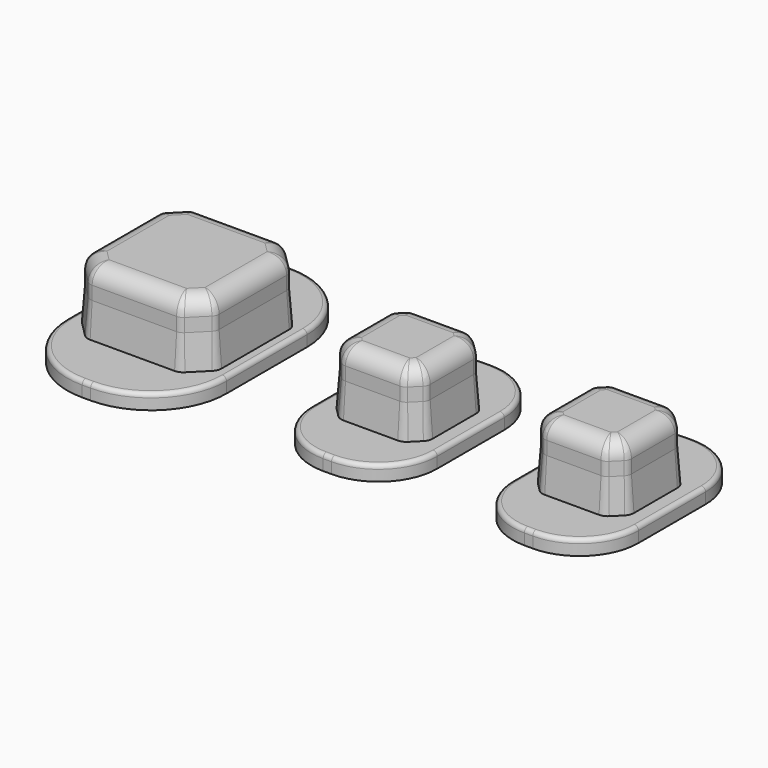
from build123d import *

# Parameters (mm, degrees)
F0_W        = 9.5
F0_H        = 15
F1_DEPTH    = 0.9
F0_W_2      = 7.5
F0_H_2      = 12
F3_DEPTH    = 3.8
F5_DEPTH    = 3.8
F6_R        = 4.5
F7_R        = 3.5
F8_SIZE     = 1.2
F9_SIZE     = 0.8
F10_R       = 1
F10_2_R     = 1
F11_R       = 0.5
F11_2_R     = 0.5
F12_SIZE2   = 2
F12_SIZE    = 0.15
F12_2_SIZE2 = 2
F12_2_SIZE  = 0.15
F14_R       = 0.25
F14_2_R     = 0.25
F14_3_R     = 0.25


with BuildPart() as f1:
    # F0 (on Top) → F1 (new body)
    with BuildSketch(Plane.XY):
        with Locations((-18.6926795918, 4.292611382)):
            Rectangle(F0_W, F0_H)
    extrude(amount=F1_DEPTH)

    # F2 (on face) → F3 (join)
    with BuildSketch(Plane.XY.offset(0.9)):
        Polygon((-14.7676795918, 8.217611382), (-22.6176795918, 8.217611382), (-22.6176795918, 4.292611382), (-22.6176795918, 0.367611382), (-18.6926795918, 0.367611382), (-14.7676795918, 0.367611382), (-14.7676795918, 4.292611382), align=None)
    extrude(amount=F3_DEPTH)

    # F6
    f6_edges = [f1.edges().sort_by_distance(p)[0] for p in [
        (-23.44268, -3.207389, 0.45),
        (-13.94268, -3.207389, 0.45),
        (-23.44268, 11.792611, 0.45),
        (-13.94268, 11.792611, 0.45),
    ]]
    fillet(f6_edges, radius=F6_R)

    # F8
    f8_edges = [f1.edges().sort_by_distance(p)[0] for p in [
        (-22.61768, 0.367611, 2.8),
        (-14.76768, 0.367611, 2.8),
        (-14.76768, 8.217611, 2.8),
        (-22.61768, 8.217611, 2.8),
    ]]
    chamfer(f8_edges, length=F8_SIZE)

    # F10
    f10_edges = [f1.edges().sort_by_distance(p)[0] for p in [
        (-14.76768, 4.292611, 4.7),
        (-15.36768, 7.617611, 4.7),
        (-15.36768, 0.967611, 4.7),
        (-18.69268, 8.217611, 4.7),
        (-18.69268, 0.367611, 4.7),
        (-22.01768, 7.617611, 4.7),
        (-22.01768, 0.967611, 4.7),
        (-22.61768, 4.292611, 4.7),
    ]]
    fillet(f10_edges, radius=F10_R)

    # F11
    f11_edges = [f1.edges().sort_by_distance(p)[0] for p in [
        (-21.41768, 0.367611, 2.3),
        (-22.61768, 1.567611, 2.3),
        (-15.96768, 0.367611, 2.3),
        (-14.76768, 1.567611, 2.3),
        (-14.76768, 7.017611, 2.3),
        (-15.96768, 8.217611, 2.3),
        (-21.41768, 8.217611, 2.3),
        (-22.61768, 7.017611, 2.3),
        (-15.060573, 6.896291, 4.407107),
        (-15.060573, 1.688932, 4.407107),
        (-16.089, 7.924718, 4.407107),
        (-16.089, 0.660505, 4.407107),
        (-21.296359, 7.924718, 4.407107),
        (-21.296359, 0.660505, 4.407107),
        (-22.324786, 6.896291, 4.407107),
        (-22.324786, 1.688932, 4.407107),
    ]]
    fillet(f11_edges, radius=F11_R)

    # F12
    f12_edges = [f1.edges().sort_by_distance(p)[0] for p in [
        (-18.69268, 0.367611, 0.9),
        (-14.76768, 4.292611, 0.9),
        (-14.80574, 7.001846, 0.9),
        (-14.80574, 1.583376, 0.9),
        (-15.36768, 0.967611, 0.9),
        (-15.36768, 7.617611, 0.9),
        (-15.983445, 0.405672, 0.9),
        (-15.983445, 8.179551, 0.9),
        (-18.69268, 8.217611, 0.9),
        (-21.401915, 0.405672, 0.9),
        (-21.401915, 8.179551, 0.9),
        (-22.01768, 0.967611, 0.9),
        (-22.01768, 7.617611, 0.9),
        (-22.579619, 1.583376, 0.9),
        (-22.579619, 7.001846, 0.9),
        (-22.61768, 4.292611, 0.9),
    ]]
    f12_side = f1.faces().sort_by_distance((-14.590127, 4.292611, 0.9))[0]
    chamfer(f12_edges, length=F12_SIZE, length2=F12_SIZE2, reference=f12_side)

    # F14
    f14_edges = [f1.edges().sort_by_distance(p)[0] for p in [
        (-22.12466, -1.889369, 0.9),
        (-18.69268, -3.207389, 0.9),
        (-15.260699, -1.889369, 0.9),
        (-23.44268, 4.292611, 0.9),
        (-13.94268, 4.292611, 0.9),
        (-22.12466, 10.474592, 0.9),
        (-15.260699, 10.474592, 0.9),
        (-18.69268, 11.792611, 0.9),
    ]]
    fillet(f14_edges, radius=F14_R)


with BuildPart() as f1b:
    # F0 (on Top) → F1, piece 2 (new body)
    with BuildSketch(Plane.XY):
        with Locations((-5.2992246673, 4.0066060089)):
            Rectangle(F0_W_2, F0_H_2)
    extrude(amount=F1_DEPTH)

    # F4 (on face) → F5 (join)
    with BuildSketch(Plane.XY.offset(0.9)):
        Polygon((-5.2992246673, 6.6316060089), (-7.9242246673, 6.6316060089), (-7.9242246673, 4.0066060089), (-7.9242246673, 1.3816060089), (-2.6742246673, 1.3816060089), (-2.6742246673, 6.6316060089), align=None)
    extrude(amount=F5_DEPTH)

    # F7
    f7_edges = [f1b.edges().sort_by_distance(p)[0] for p in [
        (-9.049225, 10.006606, 0.45),
        (-1.549225, 10.006606, 0.45),
        (-9.049225, -1.993394, 0.45),
        (-1.549225, -1.993394, 0.45),
    ]]
    fillet(f7_edges, radius=F7_R)

    # F9
    f9_edges = [f1b.edges().sort_by_distance(p)[0] for p in [
        (-7.924225, 1.381606, 2.8),
        (-2.674225, 1.381606, 2.8),
        (-7.924225, 6.631606, 2.8),
        (-2.674225, 6.631606, 2.8),
    ]]
    chamfer(f9_edges, length=F9_SIZE)

    # F10#2
    f10_2_edges = [f1b.edges().sort_by_distance(p)[0] for p in [
        (-5.299225, 6.631606, 4.7),
        (-7.524225, 6.231606, 4.7),
        (-3.074225, 6.231606, 4.7),
        (-7.924225, 4.006606, 4.7),
        (-2.674225, 4.006606, 4.7),
        (-7.524225, 1.781606, 4.7),
        (-3.074225, 1.781606, 4.7),
        (-5.299225, 1.381606, 4.7),
    ]]
    fillet(f10_2_edges, radius=F10_2_R)

    # F11#2
    f11_2_edges = [f1b.edges().sort_by_distance(p)[0] for p in [
        (-7.124225, 1.381606, 2.3),
        (-3.474225, 1.381606, 2.3),
        (-2.674225, 2.181606, 2.3),
        (-2.674225, 5.831606, 2.3),
        (-3.474225, 6.631606, 2.3),
        (-7.924225, 2.181606, 2.3),
        (-7.924225, 5.831606, 2.3),
        (-7.124225, 6.631606, 2.3),
        (-7.002904, 6.338713, 4.407107),
        (-3.595545, 6.338713, 4.407107),
        (-7.631331, 5.710286, 4.407107),
        (-2.967118, 5.710286, 4.407107),
        (-7.631331, 2.302926, 4.407107),
        (-2.967118, 2.302926, 4.407107),
        (-7.002904, 1.674499, 4.407107),
        (-3.595545, 1.674499, 4.407107),
    ]]
    fillet(f11_2_edges, radius=F11_2_R)

    # F12#2
    f12_2_edges = [f1b.edges().sort_by_distance(p)[0] for p in [
        (-5.299225, 1.381606, 0.9),
        (-7.524225, 1.781606, 0.9),
        (-7.924225, 4.006606, 0.9),
        (-3.074225, 1.781606, 0.9),
        (-2.674225, 4.006606, 0.9),
        (-3.074225, 6.231606, 0.9),
        (-5.299225, 6.631606, 0.9),
        (-7.524225, 6.231606, 0.9),
        (-7.10846, 6.593546, 0.9),
        (-3.48999, 6.593546, 0.9),
        (-2.712285, 5.815841, 0.9),
        (-7.886164, 5.815841, 0.9),
        (-2.712285, 2.197371, 0.9),
        (-7.886164, 2.197371, 0.9),
        (-3.48999, 1.419666, 0.9),
        (-7.10846, 1.419666, 0.9),
    ]]
    f12_2_side = f1b.faces().sort_by_distance((-5.299225, 6.773116, 0.9))[0]
    chamfer(f12_2_edges, length=F12_2_SIZE, length2=F12_2_SIZE2, reference=f12_2_side)


with BuildPart() as f13_1:
    # F13: copy of F1b
    add(f1b.part.moved(Location((12, 0, 0))))

    # F14#3
    f14_3_edges = [f13_1.edges().sort_by_distance(p)[0] for p in [
        (3.975902, -0.968268, 0.9),
        (6.700775, 10.006606, 0.9),
        (9.425649, 8.98148, 0.9),
        (3.975902, 8.98148, 0.9),
        (10.450775, 4.006606, 0.9),
        (2.950775, 4.006606, 0.9),
        (9.425649, -0.968268, 0.9),
        (6.700775, -1.993394, 0.9),
    ]]
    fillet(f14_3_edges, radius=F14_3_R)


with BuildPart() as f1b_1:
    add(f1b.part)

    # F14#2
    f14_2_edges = [f1b_1.edges().sort_by_distance(p)[0] for p in [
        (-8.024098, -0.968268, 0.9),
        (-5.299225, 10.006606, 0.9),
        (-2.574351, 8.98148, 0.9),
        (-8.024098, 8.98148, 0.9),
        (-1.549225, 4.006606, 0.9),
        (-9.049225, 4.006606, 0.9),
        (-2.574351, -0.968268, 0.9),
        (-5.299225, -1.993394, 0.9),
    ]]
    fillet(f14_2_edges, radius=F14_2_R)


solid = Compound([f1.part, f13_1.part, f1b_1.part])
